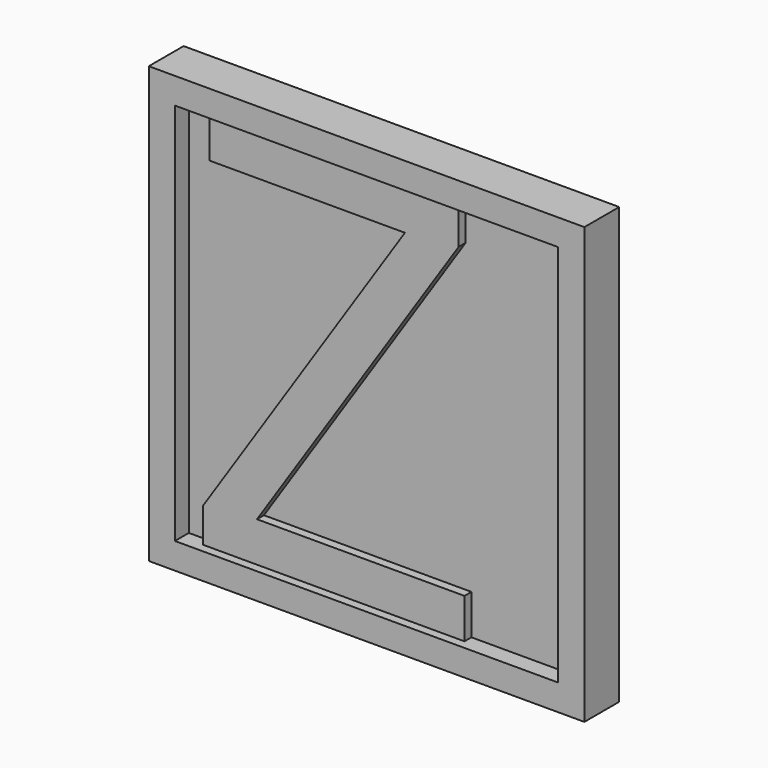
from build123d import *

# Parameters (mm, degrees)
F0_W         = 25.4
F0_H         = 25.4
F1_DEPTH     = 2.54
F2_T         = -1.524
F3_TEXT_SIZE = 31.0444444444
F4_DEPTH     = 0.508


# Not quite as in the source:
# - Text() gives the source's letters only with a copy of the font that has no kerning and outlines rounded to 1/6400 em; it was checked with that copy


with BuildPart() as f1:
    # F0 (on Front) → F1 (new body)
    with BuildSketch(Plane.XZ):
        with Locations((-11.7662722125, -14.0914778829)):
            Rectangle(F0_W, F0_H)
    extrude(amount=F1_DEPTH)

    # F2
    f2_openings = [f1.faces().sort_by_distance(p)[0] for p in [
        (-11.766272, -2.54, -14.091478),
    ]]
    offset(amount=F2_T, openings=f2_openings)

    # F3 (on face) → F4 (join)
    with BuildSketch(Plane.XZ.offset(1.524)):
        with Locations((-22.9422722125, -25.2674778829)):
            Text('Z', F3_TEXT_SIZE, font='Open Sans', text_align=(TextAlign.LEFT, TextAlign.BOTTOM))
    extrude(amount=F4_DEPTH)


solid = f1.part
